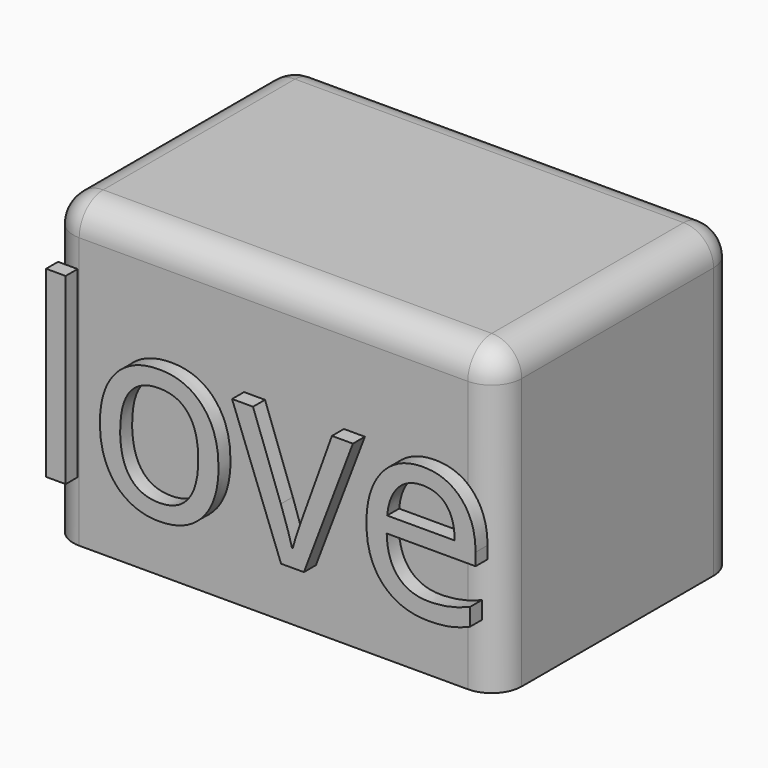
from build123d import *

# Parameters (mm, degrees)
F0_W          = 76.0191977024
F0_H          = 51.0279498994
F1_DEPTH      = 50.8
F2_R          = 5.08
F3_R          = 5.08
F4_R          = 5.08
F5_R          = 5.08
F6_TEXT_SIZE  = 44.9348260493
F7_DEPTH      = 2.54
F8_TEXT_SIZE  = 40.8791626493
F9_DEPTH      = 2.54
F10_TEXT_SIZE = 26.2233687358
F11_DEPTH     = 2.54


# Not quite as in the source:
# - Text() gives the source's letters only with a copy of the font that has no kerning and outlines rounded to 1/6400 em; it was checked with that copy


with BuildPart() as f1:
    # F0 (on Front) → F1 (new body)
    with BuildSketch(Plane.XZ):
        with Locations((38.0095988512, 25.5139749497)):
            Rectangle(F0_W, F0_H)
    extrude(amount=F1_DEPTH)

    # F2
    f2_edges = [f1.edges().sort_by_distance(p)[0] for p in [
        (38.009599, -50.8, 51.02795),
    ]]
    fillet(f2_edges, radius=F2_R)

    # F3
    f3_edges = [f1.edges().sort_by_distance(p)[0] for p in [
        (76.019198, -22.86, 51.02795),
    ]]
    fillet(f3_edges, radius=F3_R)

    # F4
    f4_edges = [f1.edges().sort_by_distance(p)[0] for p in [
        (35.469599, 0, 51.02795),
    ]]
    fillet(f4_edges, radius=F4_R)

    # F5
    f5_edges = [f1.edges().sort_by_distance(p)[0] for p in [
        (0, -25.4, 51.02795),
    ]]
    fillet(f5_edges, radius=F5_R)

    # F6 (on face) → F7 (join)
    with BuildSketch(Plane(origin=(0, 0, 0), x_dir=(0, -1, 0), z_dir=(-1, 0, 0))):
        with Locations((12.0766991749, 6.0050995089)):
            Text('I', F6_TEXT_SIZE, font='Open Sans', text_align=(TextAlign.LEFT, TextAlign.BOTTOM))
    extrude(amount=F7_DEPTH)

    # F8 (on face) → F9 (join)
    with BuildSketch(Plane.XZ.offset(50.8)):
        with Locations((-2.0134439692, 10.133292526)):
            Text('love', F8_TEXT_SIZE, font='Open Sans', text_align=(TextAlign.LEFT, TextAlign.BOTTOM))
    extrude(amount=F9_DEPTH)

    # F10 (on face) → F11 (join)
    with BuildSketch(Plane(origin=(0, 0, 0), x_dir=(-1, 0, 0), z_dir=(0, 1, 0))):
        with Locations((-62.2962042689, 16.127333045)):
            Text('you', F10_TEXT_SIZE, font='Open Sans', text_align=(TextAlign.LEFT, TextAlign.BOTTOM))
    extrude(amount=F11_DEPTH)


solid = f1.part
